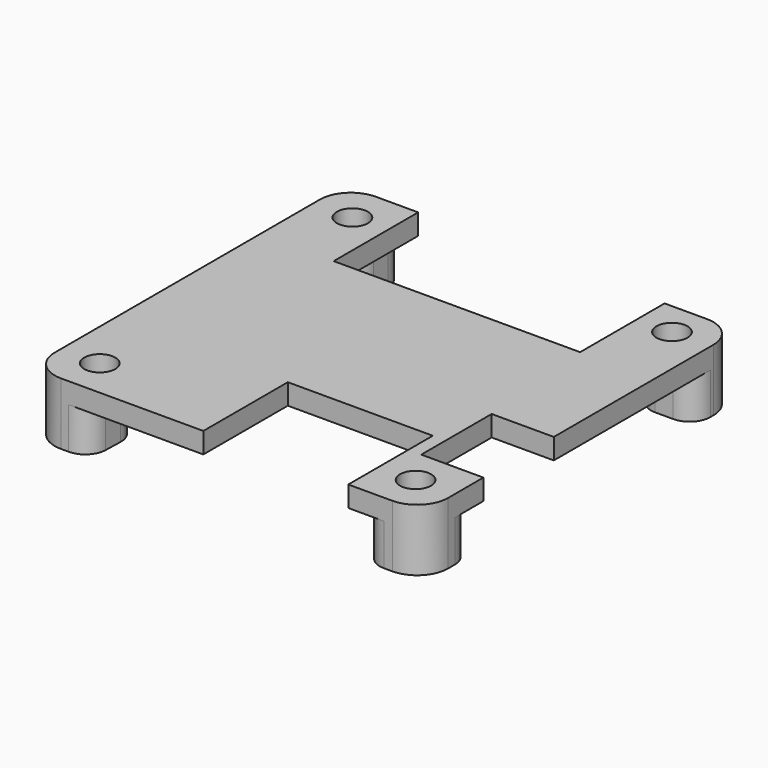
from build123d import *

# Parameters (mm, degrees)
F0_R        = 1.5
F1_DEPTH    = 2
F2_DEPTH    = 4
F3_T1_DEPTH = 9
F4_T1_DEPTH = 9
F4_T3_DEPTH = 8.8612846748


# Not quite as in the source:
# - a fillet or chamfer that OpenCascade refuses, or shapes differently, is made with other operations: its cross-section is extruded or revolved along the edge and cut away or added


with BuildPart() as f1:
    # F0 (on Top) → F1 (new body)
    with BuildSketch(Plane.XY):
        with BuildLine():
            Line((11.75, -19), (13.2, -19))
            Line((13.2, -19), (13.2, -15.25))
            ThreePointArc((13.2, -15.25), (13.8004310986, -13.8004310986), (15.25, -13.2))
            Line((15.25, -13.2), (19, -13.2))
            Line((19, -13.2), (19, -11.75))
            Line((19, -11.75), (13, -11.75))
            Line((13, -11.75), (13, -3.25))
            Line((13, -3.25), (19, -3.25))
            Line((19, -3.25), (19, 13.6544716179))
            Line((19, 13.6544716179), (15.25, 13.6544716179))
            ThreePointArc((15.25, 13.6544716179), (13.8004310986, 14.2549027165), (13.2, 15.7044716179))
            Line((13.2, 15.7044716179), (13.2, 19))
            Line((13.2, 19), (11.9, 19))
            Line((11.9, 19), (11.9, 8.8))
            Line((11.9, 8.8), (0, 8.8))
            Line((0, 8.8), (-11.9, 8.8))
            Line((-11.9, 8.8), (-11.9, 19))
            Line((-11.9, 19), (-13.2, 19))
            Line((-13.2, 19), (-13.2, 15.25))
            ThreePointArc((-13.2, 15.25), (-13.8004310986, 13.8004310986), (-15.25, 13.2))
            Line((-15.25, 13.2), (-19, 13.2))
            Line((-19, 13.2), (-19, -13.2))
            Line((-19, -13.2), (-15.25, -13.2))
            ThreePointArc((-15.25, -13.2), (-13.7801859172, -13.8209630649), (-13.2008111101, -15.3076618908))
            Line((-13.2008111101, -15.3076618908), (-13.304709388, -19))
            Line((-13.304709388, -19), (-2.25, -19))
            Line((-2.25, -19), (-2.25, -8.8))
            Line((-2.25, -8.8), (11.75, -8.8))
            Line((11.75, -8.8), (11.75, -19))
        make_face()
        with BuildLine():
            Line((-19, 16), (-19, 13.2))
            Line((-19, 13.2), (-15.25, 13.2))
            ThreePointArc((-15.25, 13.2), (-13.8004310986, 13.8004310986), (-13.2, 15.25))
            Line((-13.2, 15.25), (-13.2, 19))
            Line((-13.2, 19), (-16, 19))
            ThreePointArc((-16, 19), (-18.1213203436, 18.1213203436), (-19, 16))
        make_face()
        with Locations((-15.25, 15.25)):
            Circle(F0_R, mode=Mode.SUBTRACT)
        with BuildLine():
            Line((15.25, 13.6544716179), (19, 13.6544716179))
            Line((19, 13.6544716179), (19, 16))
            ThreePointArc((19, 16), (18.1213203436, 18.1213203436), (16, 19))
            Line((16, 19), (13.2, 19))
            Line((13.2, 19), (13.2, 15.7044716179))
            ThreePointArc((13.2, 15.7044716179), (13.8004310986, 14.2549027165), (15.25, 13.6544716179))
        make_face()
        with Locations((15.25, 15.7044716179)):
            Circle(F0_R, mode=Mode.SUBTRACT)
        with BuildLine():
            Line((13.2, -19), (16, -19))
            ThreePointArc((16, -19), (18.1213203436, -18.1213203436), (19, -16))
            Line((19, -16), (19, -13.2))
            Line((19, -13.2), (15.25, -13.2))
            ThreePointArc((15.25, -13.2), (13.8004310986, -13.8004310986), (13.2, -15.25))
            Line((13.2, -15.25), (13.2, -19))
        make_face()
        with Locations((15.25, -15.25)):
            Circle(F0_R, mode=Mode.SUBTRACT)
        with BuildLine():
            Line((-16, -19), (-13.304709388, -19))
            Line((-13.304709388, -19), (-13.2008111101, -15.3076618908))
            ThreePointArc((-13.2008111101, -15.3076618908), (-13.7801859172, -13.8209630649), (-15.25, -13.2))
            Line((-15.25, -13.2), (-19, -13.2))
            Line((-19, -13.2), (-19, -16))
            ThreePointArc((-19, -16), (-18.1213203436, -18.1213203436), (-16, -19))
        make_face()
        with Locations((-15.25, -15.25)):
            Circle(F0_R, mode=Mode.SUBTRACT)
    extrude(amount=F1_DEPTH)

    # F0 (on Top) → F2 (join)
    with BuildSketch(Plane.XY):
        with BuildLine():
            Line((-16, -19), (-13.304709388, -19))
            Line((-13.304709388, -19), (-13.2008111101, -15.3076618908))
            ThreePointArc((-13.2008111101, -15.3076618908), (-13.7801859172, -13.8209630649), (-15.25, -13.2))
            Line((-15.25, -13.2), (-19, -13.2))
            Line((-19, -13.2), (-19, -16))
            ThreePointArc((-19, -16), (-18.1213203436, -18.1213203436), (-16, -19))
        make_face()
        with Locations((-15.25, -15.25)):
            Circle(F0_R, mode=Mode.SUBTRACT)
        with BuildLine():
            Line((13.2, -19), (16, -19))
            ThreePointArc((16, -19), (18.1213203436, -18.1213203436), (19, -16))
            Line((19, -16), (19, -13.2))
            Line((19, -13.2), (15.25, -13.2))
            ThreePointArc((15.25, -13.2), (13.8004310986, -13.8004310986), (13.2, -15.25))
            Line((13.2, -15.25), (13.2, -19))
        make_face()
        with Locations((15.25, -15.25)):
            Circle(F0_R, mode=Mode.SUBTRACT)
        with BuildLine():
            Line((15.25, 13.6544716179), (19, 13.6544716179))
            Line((19, 13.6544716179), (19, 16))
            ThreePointArc((19, 16), (18.1213203436, 18.1213203436), (16, 19))
            Line((16, 19), (13.2, 19))
            Line((13.2, 19), (13.2, 15.7044716179))
            ThreePointArc((13.2, 15.7044716179), (13.8004310986, 14.2549027165), (15.25, 13.6544716179))
        make_face()
        with Locations((15.25, 15.7044716179)):
            Circle(F0_R, mode=Mode.SUBTRACT)
        with BuildLine():
            Line((-19, 16), (-19, 13.2))
            Line((-19, 13.2), (-15.25, 13.2))
            ThreePointArc((-15.25, 13.2), (-13.8004310986, 13.8004310986), (-13.2, 15.25))
            Line((-13.2, 15.25), (-13.2, 19))
            Line((-13.2, 19), (-16, 19))
            ThreePointArc((-16, 19), (-18.1213203436, 18.1213203436), (-19, 16))
        make_face()
        with Locations((-15.25, 15.25)):
            Circle(F0_R, mode=Mode.SUBTRACT)
    extrude(amount=-F2_DEPTH)

    # F3: fillet of radius 2 on 1 edges, made by hand

    # F3_s2 → F3_t1 (cut)
    with BuildSketch(Plane.XY.offset(-9)):
        with BuildLine():
            ThreePointArc((-13.2, 17), (-13.7857864376, 18.4142135624), (-15.2, 19))
            Line((-15.2, 19), (-13.2, 19))
            Line((-13.2, 19), (-13.2, 17))
        make_face()
    extrude(amount=F3_T1_DEPTH, mode=Mode.SUBTRACT)

    # F4: fillet of radius 2 on 6 edges, made by hand

    # F4_s2 → F4_t1 (cut)
    with BuildSketch(Plane.XY.offset(-9)):
        with BuildLine():
            ThreePointArc((13.2, 17), (13.7857864376, 18.4142135624), (15.2, 19))
            Line((15.2, 19), (13.2, 19))
            Line((13.2, 19), (13.2, 17))
        make_face()
        with BuildLine():
            ThreePointArc((17, 13.6544716179), (18.4142135624, 14.2402580556), (19, 15.6544716179))
            Line((19, 15.6544716179), (19, 13.6544716179))
            Line((19, 13.6544716179), (17, 13.6544716179))
        make_face()
        with BuildLine():
            ThreePointArc((17, -13.2), (18.4142135624, -13.7857864376), (19, -15.2))
            Line((19, -15.2), (19, -13.2))
            Line((19, -13.2), (17, -13.2))
        make_face()
        with BuildLine():
            ThreePointArc((13.2, -17), (13.7857864376, -18.4142135624), (15.2, -19))
            Line((15.2, -19), (13.2, -19))
            Line((13.2, -19), (13.2, -17))
        make_face()
        with BuildLine():
            ThreePointArc((-17, -13.2), (-18.4142135624, -13.7857864376), (-19, -15.2))
            Line((-19, -15.2), (-19, -13.2))
            Line((-19, -13.2), (-17, -13.2))
        make_face()
    extrude(amount=F4_T1_DEPTH, mode=Mode.SUBTRACT)

    # F4_s4 → F4_t3 (cut)
    with BuildSketch(Plane.XY.offset(-8.8612846748)):
        with BuildLine():
            ThreePointArc((-13.2500145849, -17.0562555032), (-13.8550408822, -18.4339649588), (-15.249223258, -19))
            Line((-15.249223258, -19), (-13.304709388, -19))
            Line((-13.304709388, -19), (-13.2500145849, -17.0562555032))
        make_face()
    extrude(amount=F4_T3_DEPTH, mode=Mode.SUBTRACT)


solid = f1.part
